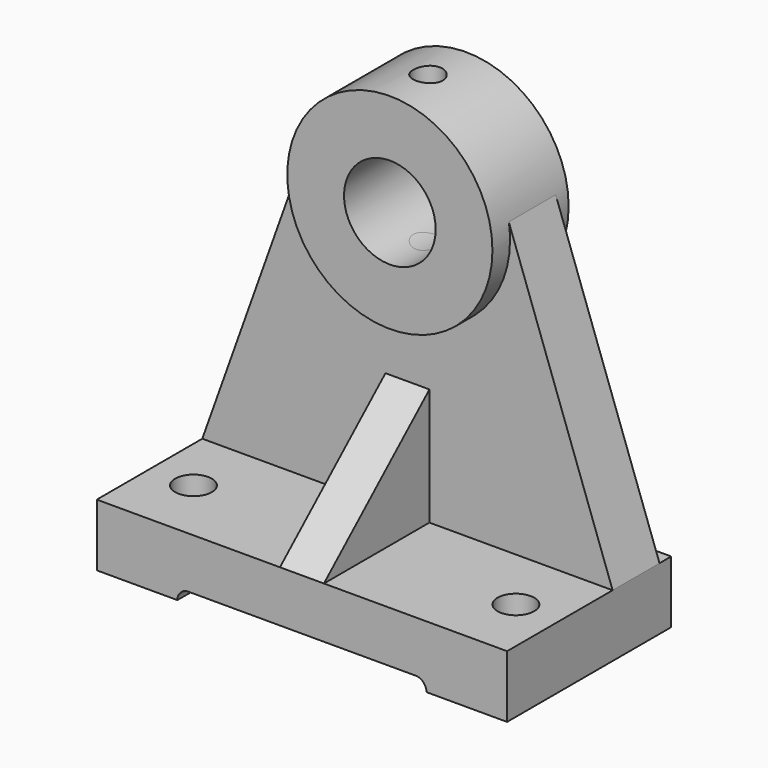
from build123d import *

# Parameters (mm, degrees)
F1_DEPTH  = 28
F3_DEPTH  = 28
F5_DEPTH  = 8
F7_DEPTH  = 4
F8_R      = 28
F9_DEPTH  = 28
F10_R     = 28
F11_DEPTH = 2
F12_R     = 12.5
F13_DEPTH = 26.001
F15_DEPTH = 112
F17_DEPTH = 50
F19_DEPTH = 50
F20_R     = 4
F21_DEPTH = 139
F22_R     = 4
F23_DEPTH = 91
F24_R     = 12.5
F25_DEPTH = 26.0010001
F26_R     = 5
F27_DEPTH = 120.0010001
F28_W     = 68
F28_H     = 3
F29_DEPTH = 28.0010001
F30_R     = 2.99999


# Not quite as in the source:
# - a fillet or chamfer is up to 0.001 mm smaller than in the source, because OpenCascade refuses the exact size


with BuildPart() as f1:
    # F0 (on Front) → F1 (new body, symmetric)
    with BuildSketch(Plane.XZ):
        Polygon((0, 17), (0, 0), (22, 0), (22, 3), (90, 3), (90, 0), (112, 0), (112, 17), align=None)
    extrude(amount=F1_DEPTH, both=True)

    # F2 (on Front) → F3 (join)
    with BuildSketch(Plane.XZ):
        with BuildLine():
            Line((28.3328655167, 96.304610259), (0, 17))
            Line((0, 17), (112, 17))
            Line((112, 17), (83.6671344833, 96.304610259))
            ThreePointArc((83.6671344833, 96.304610259), (56, 64), (28.3328655167, 96.304610259))
        make_face()
    extrude(amount=-F3_DEPTH)

    # F4 (on face) → F5 (cut)
    with BuildSketch(Plane.XZ):
        with BuildLine():
            ThreePointArc((83.6671344833, 96.304610259), (56, 64), (28.3328655167, 96.304610259))
            Line((28.3328655167, 96.304610259), (0, 17))
            Line((0, 17), (112, 17))
            Line((112, 17), (83.6671344833, 96.304610259))
        make_face()
    extrude(amount=-F5_DEPTH, mode=Mode.SUBTRACT)

    # F6 (on face) → F7 (cut)
    with BuildSketch(Plane(origin=(0, 28, 0), x_dir=(-1, 0, 0), z_dir=(0, 1, 0))):
        with BuildLine():
            Line((-83.6671344833, 96.304610259), (-112, 17))
            Line((-112, 17), (0, 17))
            Line((0, 17), (-28.3328655167, 96.304610259))
            ThreePointArc((-28.3328655167, 96.304610259), (-56, 64), (-83.6671344833, 96.304610259))
        make_face()
    extrude(amount=-F7_DEPTH, mode=Mode.SUBTRACT)

    # F8 (on Front) → F9 (join)
    with BuildSketch(Plane.XZ):
        with Locations((56, 92)):
            Circle(F8_R)
    extrude(amount=-F9_DEPTH)

    # F10 (on face) → F11 (cut)
    with BuildSketch(Plane.XZ):
        with Locations((56, 92)):
            Circle(F10_R)
    extrude(amount=-F11_DEPTH, mode=Mode.SUBTRACT)

    # F12 (on face) → F13 (cut, through all)
    with BuildSketch(Plane.XZ.offset(-2)):
        with Locations((56, 92)):
            Circle(F12_R)
    extrude(amount=-F13_DEPTH, mode=Mode.SUBTRACT)

    # F14 (on Right) → F15 (join)
    with BuildSketch(Plane.YZ):
        Polygon((8, 49), (-28, 17), (8, 17), align=None)
    extrude(amount=F15_DEPTH)

    # F16 (on face) → F17 (cut)
    with BuildSketch(Plane.YZ.offset(112)):
        Polygon((8, 49), (-28, 17), (8, 17), align=None)
    extrude(amount=-F17_DEPTH, mode=Mode.SUBTRACT)

    # F18 (on face) → F19 (cut)
    with BuildSketch(Plane(origin=(0, 0, 0), x_dir=(0, -1, 0), z_dir=(-1, 0, 0))):
        Polygon((-8, 49), (-8, 17), (28, 17), align=None)
    extrude(amount=-F19_DEPTH, mode=Mode.SUBTRACT)

    # F20 (on Top) → F21 (cut)
    with BuildSketch(Plane.XY):
        with Locations((56, 15)):
            Circle(F20_R)
    extrude(amount=F21_DEPTH, mode=Mode.SUBTRACT)

    # F22 (on Top) → F23 (join)
    with BuildSketch(Plane.XY):
        with Locations((56, 15)):
            Circle(F22_R)
    extrude(amount=F23_DEPTH)

    # F24 (on face) → F25 (cut, through all)
    with BuildSketch(Plane.XZ.offset(-2)):
        with Locations((56, 92)):
            Circle(F24_R)
    extrude(amount=-F25_DEPTH, mode=Mode.SUBTRACT)

    # F26 (on Top) → F27 (cut, through all)
    with BuildSketch(Plane.XY):
        with Locations((12, -10)):
            Circle(F26_R)
        with Locations((100, -10)):
            Circle(F26_R)
    extrude(amount=F27_DEPTH, mode=Mode.SUBTRACT)

    # F28 (on Front) → F29 (cut, through all)
    with BuildSketch(Plane.XZ):
        with Locations((56, 1.5)):
            Rectangle(F28_W, F28_H)
    extrude(amount=-F29_DEPTH, mode=Mode.SUBTRACT)

    # F30 (radius 3 in the source; OpenCascade refuses exactly that, so slightly less here)
    f30_edges = [f1.edges().sort_by_distance(p)[0] for p in [
        (90, 0, 3),
        (22, 0, 3),
    ]]
    fillet(f30_edges, radius=F30_R)


solid = f1.part
